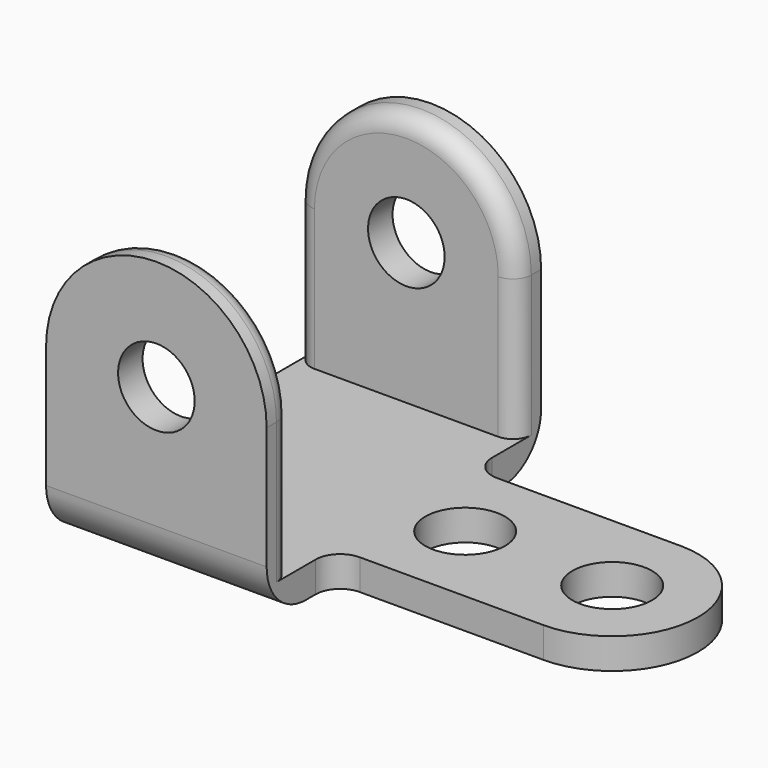
from build123d import *

# Parameters (mm, degrees)
F0_R     = 10.3251
F1_DEPTH = 7.9375
F2_R     = 6.35
F3_R     = 9.92251
F4_DEPTH = 7.9375
F6_R     = 12.7
F7_R     = 4.7625


with BuildPart() as f1:
    # F0 (on Top) → F1 (new body)
    with BuildSketch(Plane.XY):
        with BuildLine():
            Line((-53.975, -22.225), (0, -22.225))
            ThreePointArc((0, -22.225), (22.225, 0), (0, 22.225))
            Line((0, 22.225), (-53.975, 22.225))
            Line((-53.975, 22.225), (-53.975, 44.45))
            Line((-53.975, 44.45), (-111.125, 44.45))
            Line((-111.125, 44.45), (-111.125, -44.45))
            Line((-111.125, -44.45), (-53.975, -44.45))
            Line((-53.975, -44.45), (-53.975, -22.225))
        make_face()
        with Locations((-38.1, 0)):
            Circle(F0_R, mode=Mode.SUBTRACT)
        Circle(F0_R, mode=Mode.SUBTRACT)
    extrude(amount=F1_DEPTH)

    # F2
    f2_edges = [f1.edges().sort_by_distance(p)[0] for p in [
        (-53.975, -22.225, 3.96875),
        (-53.975, 22.225, 3.96875),
    ]]
    fillet(f2_edges, radius=F2_R)

    # F3 (on face) → F4 (join)
    with BuildSketch(Plane.XZ.offset(44.45)):
        with BuildLine():
            Line((-111.125, 44.45), (-111.125, 7.9375))
            Line((-111.125, 7.9375), (-53.975, 7.9375))
            Line((-53.975, 7.9375), (-53.975, 44.45))
            ThreePointArc((-53.975, 44.45), (-82.55, 73.025), (-111.125, 44.45))
        make_face()
        with Locations((-82.55, 44.45)):
            Circle(F3_R, mode=Mode.SUBTRACT)
    extrude(amount=-F4_DEPTH)

    # F5: F1 across plane


with BuildPart() as f1_1:
    add(f1.part)
    add(f1.part.mirror(Plane.XZ))

    # F6
    f6_edges = [f1_1.edges().sort_by_distance(p)[0] for p in [
        (-82.55, 44.45, 0),
        (-82.55, -44.45, 0),
    ]]
    fillet(f6_edges, radius=F6_R)

    # F7
    f7_edges = [f1_1.edges().sort_by_distance(p)[0] for p in [
        (-82.55, 36.5125, 73.025),
        (-82.55, -36.5125, 73.025),
    ]]
    fillet(f7_edges, radius=F7_R)


solid = f1_1.part
